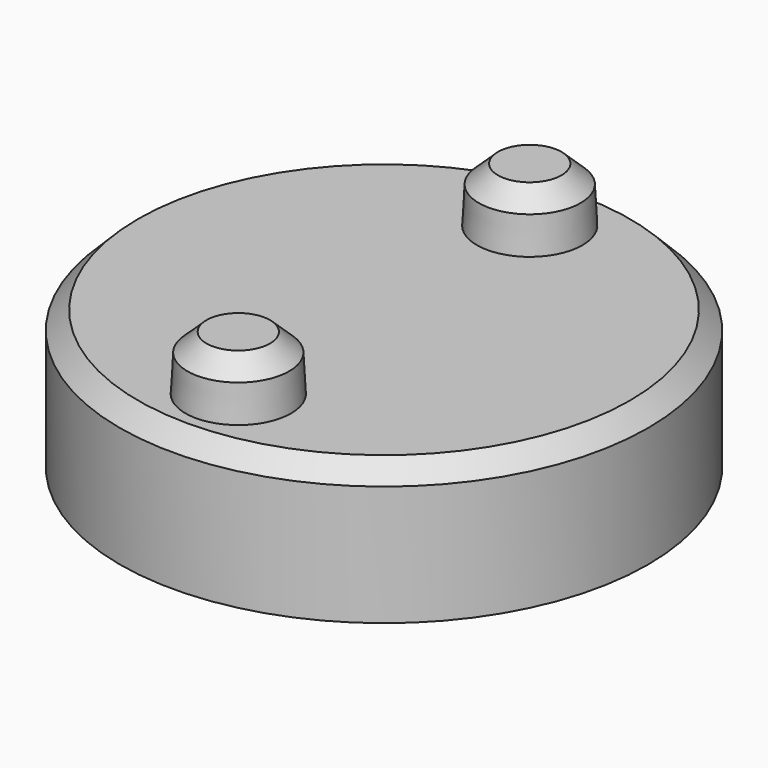
from build123d import *

# Parameters (mm, degrees)
F0_R      = 7.25
F1_DEPTH  = 3.8
F2_R      = 1.45
F3_DEPTH  = 1.5
F3_TAPER  = 3
F8_DEPTH  = 3
F10_DEPTH = 2.5
F10_TAPER = 3
F11_R     = 0.5
F12_SIZE  = 0.5


# Not quite as in the source:
# - a fillet or chamfer that OpenCascade refuses, or shapes differently, is made with other operations: its cross-section is extruded or revolved along the edge and cut away or added


with BuildPart() as f1:
    # F0 (on Top) → F1 (new body)
    with BuildSketch(Plane.XY):
        Circle(F0_R)
    extrude(amount=F1_DEPTH)

    # F2 (on face) → F3 (join)
    with BuildSketch(Plane.XY.offset(3.8)):
        with Locations((0, 5)):
            Circle(F2_R)
        with Locations((0, -5)):
            Circle(F2_R)
    extrude(amount=F3_DEPTH, taper=F3_TAPER)

    # F4: chamfer of 0.5 on 2 edges, made by hand

    # F4_s1 → F4_t2 (revolve, cut)
    with BuildSketch(Plane.XZ.offset(-5)):
        Polygon((1.3975563092, 4.8006852326), (0.8713883311, 5.3), (1.3713883311, 5.3), align=None)
    revolve(axis=Axis((0, 5, 5.3), (0, 0, -1)), mode=Mode.SUBTRACT)

    # F4_s3 → F4_t4 (revolve, cut)
    with BuildSketch(Plane.XZ.offset(5)):
        Polygon((1.3975563092, 4.8006852326), (0.8713883311, 5.3), (1.3713883311, 5.3), align=None)
    revolve(axis=Axis((0, -5, 5.3), (0, 0, -1)), mode=Mode.SUBTRACT)

    # F5 (on Right) → F6 (revolve, cut)
    with BuildSketch(Plane.YZ):
        with BuildLine():
            add(Edge.make_bspline(
                [(0, 3.2), (-3, 3.2), (-6.75, 2.5), (-6.75, 0)],
                knots=[0, 0, 0, 0, 7.4701070943, 7.4701070943, 7.4701070943, 7.4701070943], degree=3))
            Line((-6.75, 0), (0, 0))
            Line((0, 0), (0, 3.2))
        make_face()
    revolve(axis=Axis((0, 0, 2.9542176053), (0, 0, 1)), mode=Mode.SUBTRACT)

    # F7 (on face) → F8 (join)
    with BuildSketch(Plane.XY):
        with BuildLine():
            Line((-1.5, 6.5812232905), (-1.5, -6.5812232905))
            ThreePointArc((-1.5, -6.5812232905), (0, -6.75), (1.5, -6.5812232905))
            Line((1.5, -6.5812232905), (1.5, 6.5812232905))
            ThreePointArc((1.5, 6.5812232905), (0, 6.75), (-1.5, 6.5812232905))
        make_face()
    extrude(amount=F8_DEPTH)

    # F9 (on face) → F10 (cut)
    with BuildSketch(Plane(origin=(0, 0, 0), x_dir=(1, 0, 0), z_dir=(0, 0, -1))):
        with BuildLine():
            ThreePointArc((0.75, 4.25), (0, 5), (-0.75, 4.25))
            Line((-0.75, 4.25), (-0.75, -4.25))
            ThreePointArc((-0.75, -4.25), (0, -5), (0.75, -4.25))
            Line((0.75, -4.25), (0.75, 4.25))
        make_face()
    extrude(amount=-F10_DEPTH, taper=F10_TAPER, mode=Mode.SUBTRACT)

    # F11
    f11_edges = [f1.edges().sort_by_distance(p)[0] for p in [
        (0, -4.868981, 2.5),
        (-0.618981, 0, 2.5),
        (0, 4.868981, 2.5),
        (0.618981, 0, 2.5),
    ]]
    fillet(f11_edges, radius=F11_R)

    # F12
    f12_edges = [f1.edges().sort_by_distance(p)[0] for p in [
        (-7.25, 0, 3.8),
    ]]
    chamfer(f12_edges, length=F12_SIZE)


solid = f1.part
